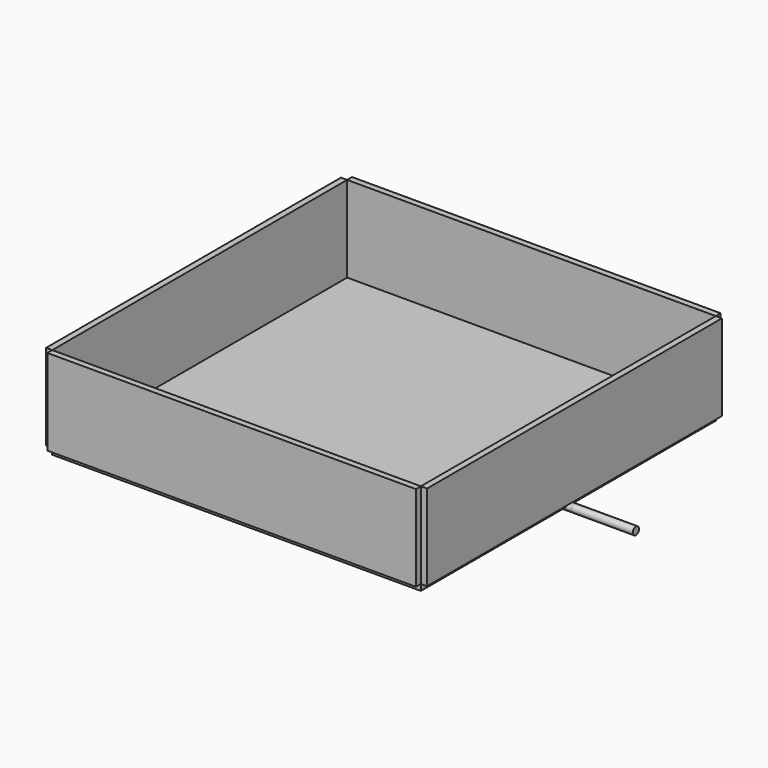
from build123d import *

# Parameters (mm, degrees)
F0_W           = 152.4
F0_H           = 152.4
F1_DEPTH       = 2.54
F2_W           = 152.4
F2_H           = 35.56
F3_DEPTH       = 2.54
F4_W           = 152.4
F4_H           = 35.56
F5_DEPTH       = 2.54
F6_W           = 152.4
F6_H           = 35.56
F7_DEPTH       = 2.54
F8_W           = 152.4
F8_H           = 35.56
F9_DEPTH       = 2.54
F10_R          = 1.5875
F11_DEPTH      = 177.8
F11_DEPTH_BACK = 25.4


with BuildPart() as f1:
    # F0 (on Top) → F1 (new body)
    with BuildSketch(Plane.XY):
        with Locations((-29.2293839186, 0.8939653635)):
            Rectangle(F0_W, F0_H)
    extrude(amount=F1_DEPTH)


with BuildPart() as f3:
    # F2 (on face) → F3 (new body)
    with BuildSketch(Plane.XZ.offset(75.3060346365)):
        with Locations((-29.2293839186, 20.32)):
            Rectangle(F2_W, F2_H)
    extrude(amount=F3_DEPTH)


with BuildPart() as f5:
    # F4 (on face) → F5 (new body)
    with BuildSketch(Plane.YZ.offset(46.9706160814)):
        with Locations((0.8939653635, 20.32)):
            Rectangle(F4_W, F4_H)
    extrude(amount=F5_DEPTH)


with BuildPart() as f7:
    # F6 (on face) → F7 (new body)
    with BuildSketch(Plane(origin=(0, 77.0939653635, 0), x_dir=(-1, 0, 0), z_dir=(0, 1, 0))):
        with Locations((29.2293839186, 20.32)):
            Rectangle(F6_W, F6_H)
    extrude(amount=F7_DEPTH)


with BuildPart() as f9:
    # F8 (on face) → F9 (new body)
    with BuildSketch(Plane(origin=(-105.4293839186, 0, 0), x_dir=(0, -1, 0), z_dir=(-1, 0, 0))):
        with Locations((-0.8939653635, 20.32)):
            Rectangle(F8_W, F8_H)
    extrude(amount=F9_DEPTH)


with BuildPart() as f11:
    # F10 (on face) → F11 (new body, two sides)
    with BuildSketch(Plane.YZ.offset(49.5106160814)) as f11_sk:
        with Locations((0.8939653635, 0)):
            Circle(F10_R)
    extrude(amount=-F11_DEPTH)
    extrude(f11_sk.sketch, amount=F11_DEPTH_BACK)


solid = Compound([f1.part, f3.part, f5.part, f7.part, f9.part, f11.part])
